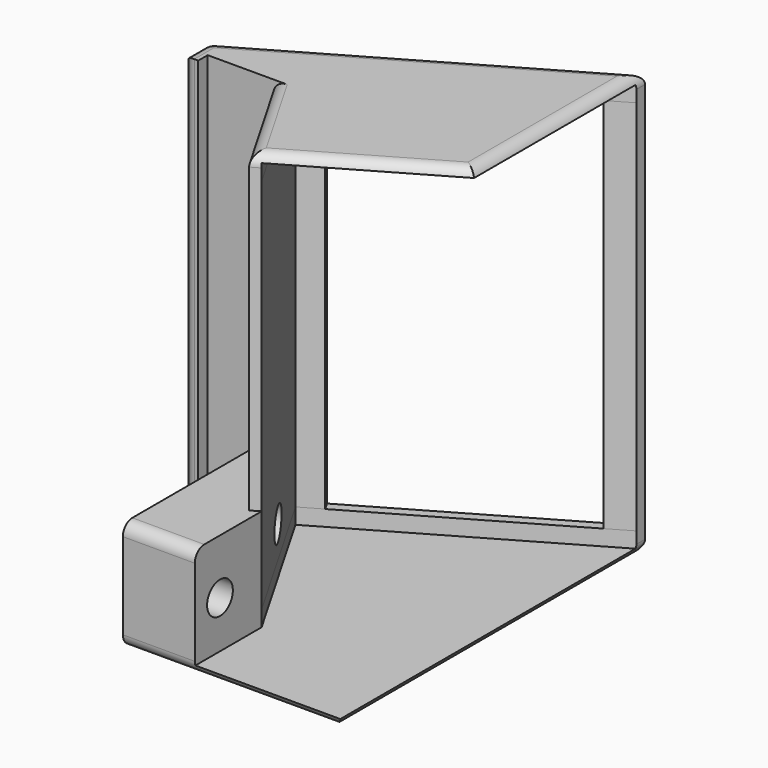
from build123d import *

# Parameters (mm, degrees)
F1_DEPTH      = 54
F2_W          = 28
F2_H          = 48
F3_DEPTH      = 50
F4_W          = 36.3328976004
F4_H          = 48
F5_DEPTH      = 3
F6_W          = 5.7282032303
F6_H          = 48
F7_DEPTH      = 20
F9_DEPTH      = 2
F11_DEPTH     = 2
F13_DEPTH     = 40
F15_DEPTH     = 13
F16_R         = 2.05
F17_DEPTH     = 25
F18_T1_DEPTH  = 46.8928601954
F18_T3_DEPTH  = 61.5
F18_T5_DEPTH  = 6.8839745962
F18_T7_DEPTH  = 30.1666666667
F18_T9_DEPTH  = 56.0044427996
F18_T11_DEPTH = 35.2128129211
F18_T13_DEPTH = 51
F18_T15_DEPTH = 16.667359312
F18_T17_DEPTH = 46.8928601954
F18_T19_DEPTH = 34.6711094662
F18_T24_DEPTH = 1.5
F18_T30_DEPTH = 1.5
F18_T36_DEPTH = 23.6658075373


# Not quite as in the source:
# - a fillet or chamfer that OpenCascade refuses, or shapes differently, is made with other operations: its cross-section is extruded or revolved along the edge and cut away or added


with BuildPart() as f1:
    # F0 (on Top) → F1 (new body)
    with BuildSketch(Plane.XY):
        Polygon((0, -1.5), (0, 0), (8.4, 0), (8.4, -24), (36.1128129211, -24), (36.1128129211, 24.5044427996), (8.4, 8.5044427996), (-2, 2.5), (-2, -1.5), align=None)
    extrude(amount=F1_DEPTH)

    # F2 (on face) → F3 (cut)
    with BuildSketch(Plane(origin=(-1.5825317547, 2.7410254038, 0), x_dir=(-0.8660254038, -0.5, 0), z_dir=(-0.5, 0.8660254038, 0))):
        with Locations((-25.5268347916, 27)):
            Rectangle(F2_W, F2_H)
    extrude(amount=-F3_DEPTH, mode=Mode.SUBTRACT)

    # F4 (on face) → F5 (cut)
    with BuildSketch(Plane(origin=(9.9825317547, 5.7634173958, 0), x_dir=(-0.5, 0.8660254038, 0), z_dir=(0.8660254038, 0.5, 0))):
        with Locations((-16.2013852907, 27)):
            Rectangle(F4_W, F4_H)
    extrude(amount=-F5_DEPTH, mode=Mode.SUBTRACT)

    # F6 (on face) → F7 (cut)
    with BuildSketch(Plane(origin=(34.2312430607, 19.7634173958, 0), x_dir=(0.5, -0.8660254038, 0), z_dir=(-0.8660254038, -0.5, 0))):
        with Locations((0.8990381057, 27)):
            Rectangle(F6_W, F6_H)
    extrude(amount=-F7_DEPTH, mode=Mode.SUBTRACT)

    # F8 (on face) → F9 (cut)
    with BuildSketch(Plane(origin=(0, 0, 51), x_dir=(1, 0, 0), z_dir=(0, 0, -1))):
        Polygon((36.1128129211, -23.1188021535), (36.1128129211, 24), (23.7023471851, 24), (6.4019237886, -5.965212315), align=None)
    extrude(amount=-F9_DEPTH, mode=Mode.SUBTRACT)

    # F10 (on face) → F11 (cut)
    with BuildSketch(Plane.XY.offset(3)):
        Polygon((36.1128129211, 23.1188021535), (6.4019237886, 5.965212315), (23.7023471851, -24), (36.1128129211, -24), align=None)
    extrude(amount=-F11_DEPTH, mode=Mode.SUBTRACT)

    # F12 (on face) → F13 (cut)
    with BuildSketch(Plane.XY.offset(54)):
        Polygon((16.4829037687, -14), (8.4, 0), (8.4, -24), (36.1128129211, -24), (36.1128129211, -2.6666666667), align=None)
    extrude(amount=-F13_DEPTH, mode=Mode.SUBTRACT)

    # F14 (on face) → F15 (cut)
    with BuildSketch(Plane.XY.offset(14)):
        Polygon((23.7023471851, -24), (17.567359312, -13.3738893001), (17.567359312, -24), align=None)
    extrude(amount=-F15_DEPTH, mode=Mode.SUBTRACT)

    # F16 (on face) → F17 (cut)
    with BuildSketch(Plane(origin=(8.4, 0, 0), x_dir=(0, -1, 0), z_dir=(-1, 0, 0))):
        with Locations((20, 7)):
            Circle(F16_R)
        with Locations((4, 7)):
            Circle(F16_R)
    extrude(amount=-F17_DEPTH, mode=Mode.SUBTRACT)

    # F18: fillet of radius 1.5 on 12 edges, made by hand

    # F18_s2 → F18_t1 (cut)
    with BuildSketch(Plane(origin=(0.3325317547, 0.1919872981, 0), x_dir=(0, 0, 1), z_dir=(0.8660254038, 0.5, 0))):
        with BuildLine():
            ThreePointArc((54, -1.6650635095), (53.5606601718, -2.7257236812), (52.5, -3.1650635095))
            Line((52.5, -3.1650635095), (54, -3.1650635095))
            Line((54, -3.1650635095), (54, -1.6650635095))
        make_face()
    extrude(amount=F18_T1_DEPTH, mode=Mode.SUBTRACT)

    # F18_s4 → F18_t3 (cut)
    with BuildSketch(Plane.XY.offset(-3.75)):
        with BuildLine():
            ThreePointArc((-0.5, -1.5), (-1.5606601718, -1.0606601718), (-2, 0))
            Line((-2, 0), (-2, -1.5))
            Line((-2, -1.5), (-0.5, -1.5))
        make_face()
    extrude(amount=F18_T3_DEPTH, mode=Mode.SUBTRACT)

    # F18_s6 → F18_t5 (cut)
    with BuildSketch(Plane.XZ.offset(-1.6339745962)):
        with BuildLine():
            ThreePointArc((-0.5, 54), (-1.5606601718, 53.5606601718), (-2, 52.5))
            Line((-2, 52.5), (-2, 54))
            Line((-2, 54), (-0.5, 54))
        make_face()
        with BuildLine():
            ThreePointArc((-0.5, 0), (-1.5606601718, 0.4393398282), (-2, 1.5))
            Line((-2, 1.5), (-2, 0))
            Line((-2, 0), (-0.5, 0))
        make_face()
    extrude(amount=F18_T5_DEPTH, mode=Mode.SUBTRACT)

    # F18_s8 → F18_t7 (cut)
    with BuildSketch(Plane(origin=(29.1775044166, 16.8456400292, 0), x_dir=(0, 0, 1), z_dir=(-0.8660254038, -0.5, 0))):
        with BuildLine():
            ThreePointArc((54, -18.8658075373), (53.5606601718, -19.9264677091), (52.5, -20.3658075373))
            Line((52.5, -20.3658075373), (54, -20.3658075373))
            Line((54, -20.3658075373), (54, -18.8658075373))
        make_face()
    extrude(amount=F18_T7_DEPTH, mode=Mode.SUBTRACT)

    # F18_s10 → F18_t9 (cut)
    with BuildSketch(Plane.XZ.offset(-28.2544427996)):
        with BuildLine():
            ThreePointArc((34.6128129211, 0), (35.6734730929, 0.4393398282), (36.1128129211, 1.5))
            Line((36.1128129211, 1.5), (36.1128129211, 0))
            Line((36.1128129211, 0), (34.6128129211, 0))
        make_face()
    extrude(amount=F18_T9_DEPTH, mode=Mode.SUBTRACT)

    # F18_s12 → F18_t11 (cut)
    with BuildSketch(Plane.YZ.offset(4.65)):
        with BuildLine():
            ThreePointArc((-22.5, 0), (-23.5606601718, 0.4393398282), (-24, 1.5))
            Line((-24, 1.5), (-24, 0))
            Line((-24, 0), (-22.5, 0))
        make_face()
    extrude(amount=F18_T11_DEPTH, mode=Mode.SUBTRACT)

    # F18_s14 → F18_t13 (cut)
    with BuildSketch(Plane.XY.offset(1.5)):
        with BuildLine():
            ThreePointArc((-2, 1.6339745962), (-1.7990381057, 2.3839745962), (-1.25, 2.9330127019))
            Line((-1.25, 2.9330127019), (-2, 2.5))
            Line((-2, 2.5), (-2, 1.6339745962))
        make_face()
    extrude(amount=F18_T13_DEPTH, mode=Mode.SUBTRACT)

    # F18_s16 → F18_t15 (cut)
    with BuildSketch(Plane.YZ.offset(4.65)):
        with BuildLine():
            ThreePointArc((-24, 12.5), (-23.5606601718, 13.5606601718), (-22.5, 14))
            Line((-22.5, 14), (-24, 14))
            Line((-24, 14), (-24, 12.5))
        make_face()
    extrude(amount=F18_T15_DEPTH, mode=Mode.SUBTRACT)

    # F18_s18 → F18_t17 (cut)
    with BuildSketch(Plane(origin=(40.94293994, 23.6384173958, 0), x_dir=(0, 0, 1), z_dir=(-0.8660254038, -0.5, 0))):
        with BuildLine():
            ThreePointArc((0, 1.6650635095), (0.4393398282, 2.7257236812), (1.5, 3.1650635095))
            Line((1.5, 3.1650635095), (0, 3.1650635095))
            Line((0, 3.1650635095), (0, 1.6650635095))
        make_face()
    extrude(amount=F18_T17_DEPTH, mode=Mode.SUBTRACT)

    # F18_s20 → F18_t19 (cut)
    with BuildSketch(Plane.XZ.offset(-28.2544427996)):
        with BuildLine():
            ThreePointArc((34.6128129211, 54), (35.6734730929, 53.5606601718), (36.1128129211, 52.5))
            Line((36.1128129211, 52.5), (36.1128129211, 54))
            Line((36.1128129211, 54), (34.6128129211, 54))
        make_face()
    extrude(amount=F18_T19_DEPTH, mode=Mode.SUBTRACT)


with BuildPart() as f18_tool22:
    # F18_s23 → F18_t24 (new body)
    with BuildSketch(Plane.XY.offset(52.5)):
        Polygon((-0.5, 1.6339745962), (-2, 1.6339745962), (-2, 2.5), (-1.25, 2.9330127019), align=None)
    extrude(amount=F18_T24_DEPTH)

    # F18_s25 → F18_t26 (revolve, cut)
    with BuildSketch(Plane(origin=(-0.5, 1.6339745962, 52.5), x_dir=(0.8660254038, -0.5, 0), z_dir=(-0.5, -0.8660254038, 0))):
        with BuildLine():
            ThreePointArc((0, -1.5), (1.5, 0), (0, 1.5))
            Line((0, 1.5), (0, -1.5))
        make_face()
    revolve(axis=Axis((-0.5, 1.6339745962, 52.5), (0, 0, 1)), mode=Mode.SUBTRACT)


with BuildPart() as f1_1:
    add(f1.part)

    # F18_t21: cut F18_tool22
    add(f18_tool22.part, mode=Mode.SUBTRACT)


with BuildPart() as f18_tool28:
    # F18_s29 → F18_t30 (new body)
    with BuildSketch(Plane.XY.offset(1.5)):
        Polygon((-0.5, 1.6339745962), (-2, 1.6339745962), (-2, 2.5), (-1.25, 2.9330127019), align=None)
    extrude(amount=-F18_T30_DEPTH)

    # F18_s31 → F18_t32 (revolve, cut)
    with BuildSketch(Plane(origin=(-0.5, 1.6339745962, 1.5), x_dir=(0.8660254038, -0.5, 0), z_dir=(0.5, 0.8660254038, 0))):
        with BuildLine():
            ThreePointArc((0, -1.5), (1.5, 0), (0, 1.5))
            Line((0, 1.5), (0, -1.5))
        make_face()
    revolve(axis=Axis((-0.5, 1.6339745962, 1.5), (0, 0, -1)), mode=Mode.SUBTRACT)


with BuildPart() as f1_2:
    add(f1_1.part)

    # F18_t27: cut F18_tool28
    add(f18_tool28.part, mode=Mode.SUBTRACT)


with BuildPart() as f18_tool34:
    # F18_s35 → F18_t36 (new body)
    with BuildSketch(Plane(origin=(12.0579037687, -20.8849019601, 0), x_dir=(0, 0, 1), z_dir=(-0.5, 0.8660254038, 0))):
        with BuildLine():
            ThreePointArc((54, 8.7746133918), (53.5606601718, 7.71395322), (52.5, 7.2746133918))
            Line((52.5, 7.2746133918), (54, 7.2746133918))
            Line((54, 7.2746133918), (54, 8.7746133918))
        make_face()
    extrude(amount=F18_T36_DEPTH)

    split(bisect_by=Plane.XZ, keep=Keep.TOP)


with BuildPart() as f1_3:
    add(f1_2.part)

    # F18_t33: cut F18_tool34
    add(f18_tool34.part, mode=Mode.SUBTRACT)


solid = f1_3.part
